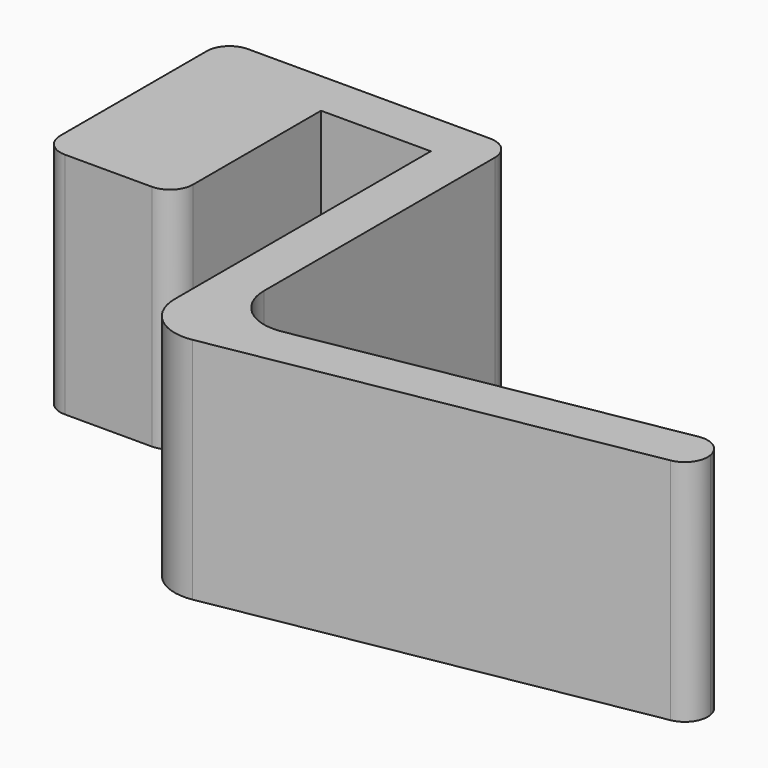
from build123d import *

# Parameters (mm, degrees)
F1_DEPTH = 25
F3_R     = 5
F4_R     = 2.49999


# Not quite as in the source:
# - a fillet or chamfer is up to 0.001 mm smaller than in the source, because OpenCascade refuses the exact size


with BuildPart() as f1:
    # F0 (on Top) → F1 (new body)
    with BuildSketch(Plane.XY):
        Polygon((0, 25), (0, 0), (14.5, 0), (14.5, 20), (26.5, 20), (26.5, -20.958767963), (80.6644264157, -11.4081181913), (79.7961855273, -6.4840794262), (31.5, -15), (31.5, 25), align=None)
    extrude(amount=F1_DEPTH)

    # F3
    f3_edges = [f1.edges().sort_by_distance(p)[0] for p in [
        (26.5, -20.958768, 12.5),
        (31.5, -15, 12.5),
    ]]
    fillet(f3_edges, radius=F3_R)

    # F4 (radius 2.5 in the source; OpenCascade refuses exactly that, so slightly less here)
    f4_edges = [f1.edges().sort_by_distance(p)[0] for p in [
        (31.5, 25, 12.5),
        (79.796186, -6.484079, 12.5),
        (80.664426, -11.408118, 12.5),
        (14.5, 0, 12.5),
        (0, 0, 12.5),
        (0, 25, 12.5),
    ]]
    fillet(f4_edges, radius=F4_R)


solid = f1.part
